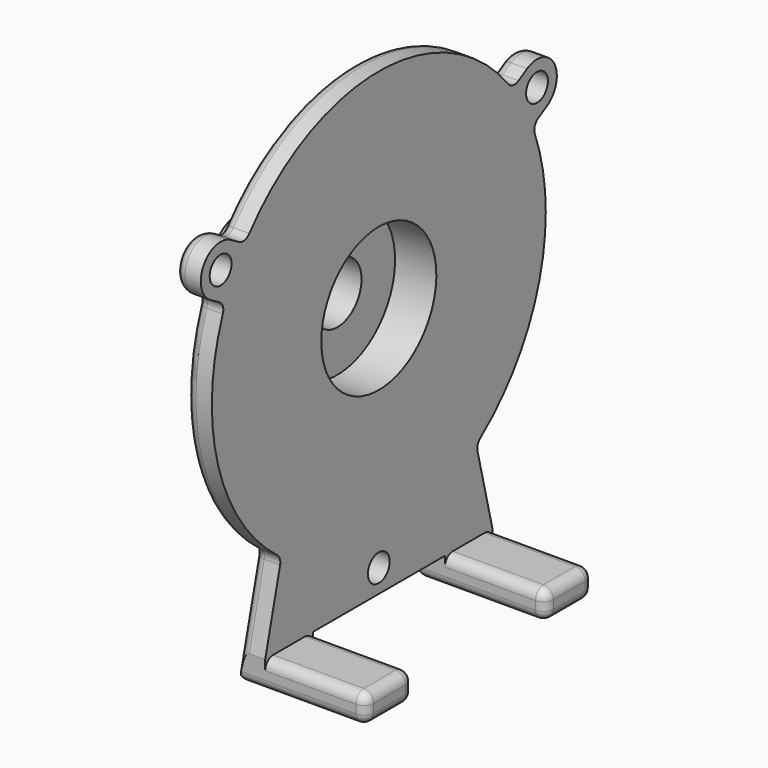
from build123d import *

# Parameters (mm, degrees)
F2_R          = 2.75
F3_DEPTH      = 5.2
F4_DEPTH      = 5.2
F5_DEPTH      = 5.2
F2_W          = 12
F2_H          = 5.7
F6_DEPTH      = 20.28
F6_DEPTH_BACK = 5.2
F7_T1_DEPTH   = 5.2
F7_T3_DEPTH   = 1.7
F7_T5_DEPTH   = 18.28
F7_T7_DEPTH   = 8
F7_T9_DEPTH   = 8
F7_T11_DEPTH  = 28.48
F7_T13_DEPTH  = 22
F7_T15_DEPTH  = 22
F7_S19_W      = 2.04
F7_S19_H      = 2.04
F7_T20_DEPTH  = 2.04
F7_S25_W      = 2.04
F7_S25_H      = 2.04
F7_T26_DEPTH  = 2.04
F7_S31_W      = 2.04
F7_S31_H      = 2.04
F7_T32_DEPTH  = 2.04
F7_S37_W      = 2.04
F7_S37_H      = 2.04
F7_T38_DEPTH  = 2.04
F7_S43_W      = 2.04
F7_S43_H      = 2.04
F7_T44_DEPTH  = 2.04
F7_S49_W      = 2.04
F7_S49_H      = 2.04
F7_T50_DEPTH  = 2.04
F7_S55_W      = 2.04
F7_S55_H      = 2.04
F7_T56_DEPTH  = 2.04
F7_S61_W      = 2.04
F7_S61_H      = 2.04
F7_T62_DEPTH  = 2.04
F7_T69_DEPTH  = 2.5190996878
F7_T71_DEPTH  = 2.5190996878
F7_T73_DEPTH  = 24.1890808372
F7_T75_DEPTH  = 24.1890808372
F7_T77_DEPTH  = 2.5190996878
F7_T79_DEPTH  = 2.5190996878
F7_T82_ANGLE  = 73.3925557793
F7_T84_ANGLE  = 101.7336044326
F7_T86_ANGLE  = 180
F7_T88_ANGLE  = 73.3925557793
F7_T90_ANGLE  = 180
F7_T92_ANGLE  = 80.8668022163
F7_T94_ANGLE  = 80.8668022163
F7_T96_ANGLE  = 66.3959416665
F7_T98_ANGLE  = 66.3959416665
F7_T100_ANGLE = 80.8668022163
F7_T102_ANGLE = 80.8668022163


# Not quite as in the source:
# - a fillet or chamfer that OpenCascade refuses, or shapes differently, is made with other operations: its cross-section is extruded or revolved along the edge and cut away or added


with BuildPart() as f1:
    # F0 (on Front) → F1 (revolve)
    with BuildSketch(Plane.XZ):
        Polygon((0, 14.51), (0, 42.1), (-5.2, 42.1), (-5.2, 20), (-10.9, 20), (-10.9, 8.925), (-28.3, 8.925), (-28.3, 6.05), (-8.33, 6.05), (-8.33, 14.51), align=None)
    revolve(axis=Axis((-6.4437054098, 0, 0), (1, 0, 0)))

    # F2 (on Right) → F3 (join, through all)
    with BuildSketch(Plane.YZ):
        with BuildLine():
            ThreePointArc((-38.7016228918, 16.5708897028), (-36.4596694993, 21.05), (-33.7016228918, 25.2311437406))
            Line((-33.7016228918, 25.2311437406), (-37.3891300983, 27.3601270189))
            ThreePointArc((-37.3891300983, 27.3601270189), (-44.2192571172, 25.53), (-42.3891300983, 18.6998729811))
            Line((-42.3891300983, 18.6998729811), (-38.7016228918, 16.5708897028))
        make_face()
        with Locations((-39.8891300983, 23.03)):
            Circle(F2_R, mode=Mode.SUBTRACT)
    extrude(amount=-F3_DEPTH)

    # F2 (on Right) → F4 (join, through all)
    with BuildSketch(Plane.YZ):
        with BuildLine():
            Line((38.7016228918, 16.5708897028), (42.3891300983, 18.6998729811))
            ThreePointArc((42.3891300983, 18.6998729811), (44.2192571172, 25.53), (37.3891300983, 27.3601270189))
            Line((37.3891300983, 27.3601270189), (33.7016228918, 25.2311437406))
            ThreePointArc((33.7016228918, 25.2311437406), (36.4596694993, 21.05), (38.7016228918, 16.5708897028))
        make_face()
        with Locations((39.8891300983, 23.03)):
            Circle(F2_R, mode=Mode.SUBTRACT)
    extrude(amount=-F4_DEPTH)

    # F2 (on Right) → F5 (join, through all)
    with BuildSketch(Plane.YZ):
        with BuildLine():
            ThreePointArc((24.57, -34.1866216523), (0, -42.1), (-24.57, -34.1866216523))
            Line((-24.57, -34.1866216523), (-28.65, -50.71))
            Line((-28.65, -50.71), (-16.65, -50.71))
            Line((-16.65, -50.71), (16.65, -50.71))
            Line((16.65, -50.71), (28.65, -50.71))
            Line((28.65, -50.71), (24.57, -34.1866216523))
        make_face()
        with Locations((0, -46.06)):
            Circle(F2_R, mode=Mode.SUBTRACT)
    extrude(amount=-F5_DEPTH)

    # F2 (on Right) → F6 (join, two sides)
    with BuildSketch(Plane.YZ) as f6_sk:
        with Locations((-22.65, -53.56)):
            Rectangle(F2_W, F2_H)
        with Locations((22.65, -53.56)):
            Rectangle(F2_W, F2_H)
    extrude(amount=F6_DEPTH)
    extrude(f6_sk.sketch, amount=-F6_DEPTH_BACK)

    # F7: fillet of radius 2 on 39 edges, made by hand

    # F7_s2 → F7_t1 (join)
    with BuildSketch(Plane.YZ.offset(-5.2)):
        with BuildLine():
            ThreePointArc((-32.6561640609, 26.5703772804), (-33.8453407807, 25.8656958459), (-35.207525774, 26.100577175))
            Line((-35.207525774, 26.100577175), (-33.7016228918, 25.2311437406))
            ThreePointArc((-33.7016228918, 25.2311437406), (-33.1856498947, 25.9060348387), (-32.6561640609, 26.5703772804))
        make_face()
        with BuildLine():
            ThreePointArc((-40.207525774, 17.4403231372), (-39.3230200794, 16.3780769929), (-39.3387037435, 14.9958790267))
            ThreePointArc((-39.3387037435, 14.9958790267), (-39.028109229, 15.7865984306), (-38.7016228918, 16.5708897028))
            Line((-38.7016228918, 16.5708897028), (-40.207525774, 17.4403231372))
        make_face()
        with BuildLine():
            ThreePointArc((32.6561640609, 26.5703772804), (33.8453407807, 25.8656958459), (35.207525774, 26.100577175))
            Line((35.207525774, 26.100577175), (33.7016228918, 25.2311437406))
            ThreePointArc((33.7016228918, 25.2311437406), (33.1856498947, 25.9060348387), (32.6561640609, 26.5703772804))
        make_face()
        with BuildLine():
            ThreePointArc((39.3387037435, 14.9958790267), (39.3230200794, 16.3780769929), (40.207525774, 17.4403231372))
            Line((40.207525774, 17.4403231372), (38.7016228918, 16.5708897028))
            ThreePointArc((38.7016228918, 16.5708897028), (39.028109229, 15.7865984306), (39.3387037435, 14.9958790267))
        make_face()
        with BuildLine():
            ThreePointArc((24.8889675585, -35.4783916643), (24.9433690993, -34.3370017965), (25.6138407126, -33.4116920246))
            ThreePointArc((25.6138407126, -33.4116920246), (25.0949117582, -33.8031862973), (24.57, -34.1866216523))
            Line((24.57, -34.1866216523), (24.8889675585, -35.4783916643))
        make_face()
        with BuildLine():
            ThreePointArc((-25.6138407126, -33.4116920246), (-24.9433690993, -34.3370017965), (-24.8889675585, -35.4783916643))
            Line((-24.8889675585, -35.4783916643), (-24.57, -34.1866216523))
            ThreePointArc((-24.57, -34.1866216523), (-25.0949117582, -33.8031862973), (-25.6138407126, -33.4116920246))
        make_face()
    extrude(amount=F7_T1_DEPTH)

    # F7_s4 → F7_t3 (cut)
    with BuildSketch(Plane.XY.offset(-54.41)):
        with BuildLine():
            ThreePointArc((18.28, -28.65), (19.6942135624, -28.0642135624), (20.28, -26.65))
            Line((20.28, -26.65), (20.28, -28.65))
            Line((20.28, -28.65), (18.28, -28.65))
        make_face()
        with BuildLine():
            ThreePointArc((18.28, -16.65), (19.6942135624, -17.2357864376), (20.28, -18.65))
            Line((20.28, -18.65), (20.28, -16.65))
            Line((20.28, -16.65), (18.28, -16.65))
        make_face()
        with BuildLine():
            ThreePointArc((18.28, 16.65), (19.6942135624, 17.2357864376), (20.28, 18.65))
            Line((20.28, 18.65), (20.28, 16.65))
            Line((20.28, 16.65), (18.28, 16.65))
        make_face()
        with BuildLine():
            ThreePointArc((18.28, 28.65), (19.6942135624, 28.0642135624), (20.28, 26.65))
            Line((20.28, 26.65), (20.28, 28.65))
            Line((20.28, 28.65), (18.28, 28.65))
        make_face()
    extrude(amount=F7_T3_DEPTH, mode=Mode.SUBTRACT)

    # F7_s6 → F7_t5 (cut)
    with BuildSketch(Plane.YZ):
        with BuildLine():
            ThreePointArc((-28.65, -52.71), (-28.0642135624, -51.2957864376), (-26.65, -50.71))
            Line((-26.65, -50.71), (-28.65, -50.71))
            Line((-28.65, -50.71), (-28.65, -52.71))
        make_face()
        with BuildLine():
            ThreePointArc((-16.65, -52.71), (-17.2357864376, -51.2957864376), (-18.65, -50.71))
            Line((-18.65, -50.71), (-16.65, -50.71))
            Line((-16.65, -50.71), (-16.65, -52.71))
        make_face()
        with BuildLine():
            ThreePointArc((16.65, -52.71), (17.2357864376, -51.2957864376), (18.65, -50.71))
            Line((18.65, -50.71), (16.65, -50.71))
            Line((16.65, -50.71), (16.65, -52.71))
        make_face()
        with BuildLine():
            ThreePointArc((28.65, -52.71), (28.0642135624, -51.2957864376), (26.65, -50.71))
            Line((26.65, -50.71), (28.65, -50.71))
            Line((28.65, -50.71), (28.65, -52.71))
        make_face()
    extrude(amount=F7_T5_DEPTH, mode=Mode.SUBTRACT)

    # F7_s8 → F7_t7 (cut)
    with BuildSketch(Plane.XZ.offset(18.65)):
        with BuildLine():
            ThreePointArc((18.28, -50.71), (19.6942135624, -51.2957864376), (20.28, -52.71))
            Line((20.28, -52.71), (20.28, -50.71))
            Line((20.28, -50.71), (18.28, -50.71))
        make_face()
        with BuildLine():
            ThreePointArc((18.28, -56.41), (19.6942135624, -55.8242135624), (20.28, -54.41))
            Line((20.28, -54.41), (20.28, -56.41))
            Line((20.28, -56.41), (18.28, -56.41))
        make_face()
    extrude(amount=F7_T7_DEPTH, mode=Mode.SUBTRACT)

    # F7_s10 → F7_t9 (cut)
    with BuildSketch(Plane.XZ.offset(-26.65)):
        with BuildLine():
            ThreePointArc((18.28, -50.71), (19.6942135624, -51.2957864376), (20.28, -52.71))
            Line((20.28, -52.71), (20.28, -50.71))
            Line((20.28, -50.71), (18.28, -50.71))
        make_face()
        with BuildLine():
            ThreePointArc((18.28, -56.41), (19.6942135624, -55.8242135624), (20.28, -54.41))
            Line((20.28, -54.41), (20.28, -56.41))
            Line((20.28, -56.41), (18.28, -56.41))
        make_face()
    extrude(amount=F7_T9_DEPTH, mode=Mode.SUBTRACT)

    # F7_s12 → F7_t11 (cut)
    with BuildSketch(Plane.YZ.offset(-10.2)):
        with BuildLine():
            ThreePointArc((-28.65, -54.41), (-28.0642135624, -55.8242135624), (-26.65, -56.41))
            Line((-26.65, -56.41), (-28.65, -56.41))
            Line((-28.65, -56.41), (-28.65, -54.41))
        make_face()
        with BuildLine():
            ThreePointArc((26.65, -56.41), (28.0642135624, -55.8242135624), (28.65, -54.41))
            Line((28.65, -54.41), (28.65, -56.41))
            Line((28.65, -56.41), (26.65, -56.41))
        make_face()
        with BuildLine():
            ThreePointArc((16.65, -54.41), (17.2357864376, -55.8242135624), (18.65, -56.41))
            Line((18.65, -56.41), (16.65, -56.41))
            Line((16.65, -56.41), (16.65, -54.41))
        make_face()
        with BuildLine():
            ThreePointArc((-18.65, -56.41), (-17.2357864376, -55.8242135624), (-16.65, -54.41))
            Line((-16.65, -54.41), (-16.65, -56.41))
            Line((-16.65, -56.41), (-18.65, -56.41))
        make_face()
    extrude(amount=F7_T11_DEPTH, mode=Mode.SUBTRACT)

    # F7_s14 → F7_t13 (cut)
    with BuildSketch(Plane.XZ.offset(11.65)):
        with BuildLine():
            ThreePointArc((-5.2, -54.41), (-4.6142135624, -55.8242135624), (-3.2, -56.41))
            Line((-3.2, -56.41), (-5.2, -56.41))
            Line((-5.2, -56.41), (-5.2, -54.41))
        make_face()
    extrude(amount=F7_T13_DEPTH, mode=Mode.SUBTRACT)

    # F7_s16 → F7_t15 (cut)
    with BuildSketch(Plane.XZ.offset(-33.65)):
        with BuildLine():
            ThreePointArc((-5.2, -54.41), (-4.6142135624, -55.8242135624), (-3.2, -56.41))
            Line((-3.2, -56.41), (-5.2, -56.41))
            Line((-5.2, -56.41), (-5.2, -54.41))
        make_face()
    extrude(amount=F7_T15_DEPTH, mode=Mode.SUBTRACT)


with BuildPart() as f7_tool18:
    # F7_s19 → F7_t20 (new body)
    with BuildSketch(Plane.YZ.offset(18.28)):
        with Locations((-27.67, -51.69)):
            Rectangle(F7_S19_W, F7_S19_H)
    extrude(amount=F7_T20_DEPTH)

    # F7_s21 → F7_t22 (revolve, cut)
    with BuildSketch(Plane(origin=(18.28, -26.65, -52.71), x_dir=(0, 0.7071067812, -0.7071067812), z_dir=(0, -0.7071067812, -0.7071067812))):
        with BuildLine():
            ThreePointArc((0, -2), (2, 0), (0, 2))
            Line((0, 2), (0, -2))
        make_face()
    revolve(axis=Axis((18.28, -26.65, -52.71), (1, 0, 0)), mode=Mode.SUBTRACT)


with BuildPart() as f1_1:
    add(f1.part)

    # F7_t17: cut F7_tool18
    add(f7_tool18.part, mode=Mode.SUBTRACT)


with BuildPart() as f7_tool24:
    # F7_s25 → F7_t26 (new body)
    with BuildSketch(Plane.XY.offset(-54.41)):
        with Locations((19.3, -27.67)):
            Rectangle(F7_S25_W, F7_S25_H)
    extrude(amount=-F7_T26_DEPTH)

    # F7_s27 → F7_t28 (revolve, cut)
    with BuildSketch(Plane(origin=(18.28, -26.65, -54.41), x_dir=(-0.7071067812, 0.7071067812, 0), z_dir=(-0.7071067812, -0.7071067812, 0))):
        with BuildLine():
            ThreePointArc((0, -2), (2, 0), (0, 2))
            Line((0, 2), (0, -2))
        make_face()
    revolve(axis=Axis((18.28, -26.65, -54.41), (0, 0, -1)), mode=Mode.SUBTRACT)


with BuildPart() as f1_2:
    add(f1_1.part)

    # F7_t23: cut F7_tool24
    add(f7_tool24.part, mode=Mode.SUBTRACT)


with BuildPart() as f7_tool30:
    # F7_s31 → F7_t32 (new body)
    with BuildSketch(Plane.XY.offset(-54.41)):
        with Locations((19.3, -17.63)):
            Rectangle(F7_S31_W, F7_S31_H)
    extrude(amount=-F7_T32_DEPTH)

    # F7_s33 → F7_t34 (revolve, cut)
    with BuildSketch(Plane(origin=(18.28, -18.65, -54.41), x_dir=(-0.7071067812, -0.7071067812, 0), z_dir=(0.7071067812, -0.7071067812, 0))):
        with BuildLine():
            ThreePointArc((0, -2), (2, 0), (0, 2))
            Line((0, 2), (0, -2))
        make_face()
    revolve(axis=Axis((18.28, -18.65, -54.41), (0, 0, -1)), mode=Mode.SUBTRACT)


with BuildPart() as f1_3:
    add(f1_2.part)

    # F7_t29: cut F7_tool30
    add(f7_tool30.part, mode=Mode.SUBTRACT)


with BuildPart() as f7_tool36:
    # F7_s37 → F7_t38 (new body)
    with BuildSketch(Plane.XZ.offset(18.65)):
        with Locations((19.3, -51.69)):
            Rectangle(F7_S37_W, F7_S37_H)
    extrude(amount=-F7_T38_DEPTH)

    # F7_s39 → F7_t40 (revolve, cut)
    with BuildSketch(Plane(origin=(18.28, -18.65, -52.71), x_dir=(-0.7071067812, 0, -0.7071067812), z_dir=(0.7071067812, 0, -0.7071067812))):
        with BuildLine():
            ThreePointArc((0, -2), (2, 0), (0, 2))
            Line((0, 2), (0, -2))
        make_face()
    revolve(axis=Axis((18.28, -18.65, -52.71), (0, 1, 0)), mode=Mode.SUBTRACT)


with BuildPart() as f1_4:
    add(f1_3.part)

    # F7_t35: cut F7_tool36
    add(f7_tool36.part, mode=Mode.SUBTRACT)


with BuildPart() as f7_tool42:
    # F7_s43 → F7_t44 (new body)
    with BuildSketch(Plane.XZ.offset(-18.65)):
        with Locations((19.3, -51.69)):
            Rectangle(F7_S43_W, F7_S43_H)
    extrude(amount=F7_T44_DEPTH)

    # F7_s45 → F7_t46 (revolve, cut)
    with BuildSketch(Plane(origin=(18.28, 18.65, -52.71), x_dir=(-0.7071067812, 0, -0.7071067812), z_dir=(-0.7071067812, 0, 0.7071067812))):
        with BuildLine():
            ThreePointArc((0, -2), (2, 0), (0, 2))
            Line((0, 2), (0, -2))
        make_face()
    revolve(axis=Axis((18.28, 18.65, -52.71), (0, -1, 0)), mode=Mode.SUBTRACT)


with BuildPart() as f1_5:
    add(f1_4.part)

    # F7_t41: cut F7_tool42
    add(f7_tool42.part, mode=Mode.SUBTRACT)


with BuildPart() as f7_tool48:
    # F7_s49 → F7_t50 (new body)
    with BuildSketch(Plane.XZ.offset(-18.65)):
        with Locations((19.3, -55.43)):
            Rectangle(F7_S49_W, F7_S49_H)
    extrude(amount=F7_T50_DEPTH)

    # F7_s51 → F7_t52 (revolve, cut)
    with BuildSketch(Plane(origin=(18.28, 18.65, -54.41), x_dir=(-0.7071067812, 0, 0.7071067812), z_dir=(0.7071067812, 0, 0.7071067812))):
        with BuildLine():
            ThreePointArc((0, -2), (2, 0), (0, 2))
            Line((0, 2), (0, -2))
        make_face()
    revolve(axis=Axis((18.28, 18.65, -54.41), (0, -1, 0)), mode=Mode.SUBTRACT)


with BuildPart() as f1_6:
    add(f1_5.part)

    # F7_t47: cut F7_tool48
    add(f7_tool48.part, mode=Mode.SUBTRACT)


with BuildPart() as f7_tool54:
    # F7_s55 → F7_t56 (new body)
    with BuildSketch(Plane.YZ.offset(18.28)):
        with Locations((27.67, -55.43)):
            Rectangle(F7_S55_W, F7_S55_H)
    extrude(amount=F7_T56_DEPTH)

    # F7_s57 → F7_t58 (revolve, cut)
    with BuildSketch(Plane(origin=(18.28, 26.65, -54.41), x_dir=(0, -0.7071067812, 0.7071067812), z_dir=(0, 0.7071067812, 0.7071067812))):
        with BuildLine():
            ThreePointArc((0, -2), (2, 0), (0, 2))
            Line((0, 2), (0, -2))
        make_face()
    revolve(axis=Axis((18.28, 26.65, -54.41), (1, 0, 0)), mode=Mode.SUBTRACT)


with BuildPart() as f1_7:
    add(f1_6.part)

    # F7_t53: cut F7_tool54
    add(f7_tool54.part, mode=Mode.SUBTRACT)


with BuildPart() as f7_tool60:
    # F7_s61 → F7_t62 (new body)
    with BuildSketch(Plane.YZ.offset(18.28)):
        with Locations((27.67, -51.69)):
            Rectangle(F7_S61_W, F7_S61_H)
    extrude(amount=F7_T62_DEPTH)

    # F7_s63 → F7_t64 (revolve, cut)
    with BuildSketch(Plane(origin=(18.28, 26.65, -52.71), x_dir=(0, -0.7071067812, -0.7071067812), z_dir=(0, -0.7071067812, 0.7071067812))):
        with BuildLine():
            ThreePointArc((0, -2), (2, 0), (0, 2))
            Line((0, 2), (0, -2))
        make_face()
    revolve(axis=Axis((18.28, 26.65, -52.71), (1, 0, 0)), mode=Mode.SUBTRACT)


with BuildPart() as f1_8:
    add(f1_7.part)

    # F7_t59: cut F7_tool60
    add(f7_tool60.part, mode=Mode.SUBTRACT)

    # F7_s65 → F7_t66 (revolve, cut)
    with BuildSketch(Plane.XZ):
        with BuildLine():
            ThreePointArc((-10.9, 18), (-10.3142135624, 19.4142135624), (-8.9, 20))
            Line((-8.9, 20), (-10.9, 20))
            Line((-10.9, 20), (-10.9, 18))
        make_face()
    revolve(axis=Axis((-10.9, 0, 0), (1, 0, 0)), mode=Mode.SUBTRACT)

    # F7_s67 → F7_t68 (revolve, cut)
    with BuildSketch(Plane.XZ):
        with BuildLine():
            ThreePointArc((-28.3, 6.925), (-27.7142135624, 8.3392135624), (-26.3, 8.925))
            Line((-26.3, 8.925), (-28.3, 8.925))
            Line((-28.3, 8.925), (-28.3, 6.925))
        make_face()
    revolve(axis=Axis((-28.3, 0, 0), (1, 0, 0)), mode=Mode.SUBTRACT)

    # F7_s70 → F7_t69 (cut)
    with BuildSketch(Plane(origin=(0, -37.707525774, 21.7704501561), x_dir=(1, 0, 0), z_dir=(0, -0.8660254038, 0.5))):
        with BuildLine():
            ThreePointArc((-3.2, 5), (-4.6142135624, 4.4142135624), (-5.2, 3))
            Line((-5.2, 3), (-5.2, 5))
            Line((-5.2, 5), (-3.2, 5))
        make_face()
    extrude(amount=F7_T69_DEPTH, mode=Mode.SUBTRACT)

    # F7_s72 → F7_t71 (cut)
    with BuildSketch(Plane(origin=(0, -39.8891300983, 23.03), x_dir=(1, 0, 0), z_dir=(0, 0.8660254038, -0.5))):
        with BuildLine():
            ThreePointArc((-3.2, 5), (-4.6142135624, 4.4142135624), (-5.2, 3))
            Line((-5.2, 3), (-5.2, 5))
            Line((-5.2, 5), (-3.2, 5))
        make_face()
    extrude(amount=F7_T71_DEPTH, mode=Mode.SUBTRACT)

    # F7_s74 → F7_t73 (cut)
    with BuildSketch(Plane(origin=(0, -9.6872865146, -39.2320343731), x_dir=(1, 0, 0), z_dir=(0, -0.2397229309, -0.9708413446))):
        with BuildLine():
            ThreePointArc((-3.2, 15.6582546967), (-4.6142135624, 15.072468259), (-5.2, 13.6582546967))
            Line((-5.2, 13.6582546967), (-5.2, 15.6582546967))
            Line((-5.2, 15.6582546967), (-3.2, 15.6582546967))
        make_face()
    extrude(amount=F7_T73_DEPTH, mode=Mode.SUBTRACT)

    # F7_s76 → F7_t75 (cut)
    with BuildSketch(Plane(origin=(0, 15.4859638688, -62.7157941379), x_dir=(1, 0, 0), z_dir=(0, -0.2397229309, 0.9708413446))):
        with BuildLine():
            ThreePointArc((-3.2, 15.6582546967), (-4.6142135624, 15.072468259), (-5.2, 13.6582546967))
            Line((-5.2, 13.6582546967), (-5.2, 15.6582546967))
            Line((-5.2, 15.6582546967), (-3.2, 15.6582546967))
        make_face()
    extrude(amount=F7_T75_DEPTH, mode=Mode.SUBTRACT)

    # F7_s78 → F7_t77 (cut)
    with BuildSketch(Plane(origin=(0, 37.707525774, 21.7704501561), x_dir=(1, 0, 0), z_dir=(0, 0.8660254038, 0.5))):
        with BuildLine():
            ThreePointArc((-3.2, 5), (-4.6142135624, 4.4142135624), (-5.2, 3))
            Line((-5.2, 3), (-5.2, 5))
            Line((-5.2, 5), (-3.2, 5))
        make_face()
    extrude(amount=F7_T77_DEPTH, mode=Mode.SUBTRACT)

    # F7_s80 → F7_t79 (cut)
    with BuildSketch(Plane(origin=(0, 39.8891300983, 23.03), x_dir=(1, 0, 0), z_dir=(0, -0.8660254038, -0.5))):
        with BuildLine():
            ThreePointArc((-3.2, 5), (-4.6142135624, 4.4142135624), (-5.2, 3))
            Line((-5.2, 3), (-5.2, 5))
            Line((-5.2, 5), (-3.2, 5))
        make_face()
    extrude(amount=F7_T79_DEPTH, mode=Mode.SUBTRACT)

    # F7_s81 → F7_t82 (revolve, cut)
    with BuildSketch(Plane(origin=(0, 0, 0), x_dir=(1, 0, 0), z_dir=(0, 0.7936268889, -0.6084047675))):
        with BuildLine():
            ThreePointArc((-3.2, 42.1), (-4.6142135624, 41.5142135624), (-5.2, 40.1))
            Line((-5.2, 40.1), (-5.2, 42.1))
            Line((-5.2, 42.1), (-3.2, 42.1))
        make_face()
    revolve(axis=Axis((-5.2, 0, 0), (-1, 0, 0)), revolution_arc=F7_T82_ANGLE, mode=Mode.SUBTRACT)

    # F7_s83 → F7_t84 (revolve, cut)
    with BuildSketch(Plane(origin=(0, 0, 0), x_dir=(1, 0, 0), z_dir=(0, -0.6311253511, -0.7756808566))):
        with BuildLine():
            ThreePointArc((-3.2, 42.1), (-4.6142135624, 41.5142135624), (-5.2, 40.1))
            Line((-5.2, 40.1), (-5.2, 42.1))
            Line((-5.2, 42.1), (-3.2, 42.1))
        make_face()
    revolve(axis=Axis((-5.2, 0, 0), (-1, 0, 0)), revolution_arc=F7_T84_ANGLE, mode=Mode.SUBTRACT)

    # F7_s85 → F7_t86 (revolve, cut)
    with BuildSketch(Plane(origin=(0, -39.8891300983, 23.03), x_dir=(1, 0, 0), z_dir=(0, 0.8660254038, -0.5))):
        with BuildLine():
            ThreePointArc((-3.2, -5), (-4.6142135624, -4.4142135624), (-5.2, -3))
            Line((-5.2, -3), (-5.2, -5))
            Line((-5.2, -5), (-3.2, -5))
        make_face()
    revolve(axis=Axis((-5.2, -39.8891300983, 23.03), (1, 0, 0)), revolution_arc=F7_T86_ANGLE, mode=Mode.SUBTRACT)

    # F7_s87 → F7_t88 (revolve, cut)
    with BuildSketch(Plane(origin=(0, 0, 0), x_dir=(1, 0, 0), z_dir=(0, -0.3561966515, 0.9344110153))):
        with BuildLine():
            ThreePointArc((-3.2, 42.1), (-4.6142135624, 41.5142135624), (-5.2, 40.1))
            Line((-5.2, 40.1), (-5.2, 42.1))
            Line((-5.2, 42.1), (-3.2, 42.1))
        make_face()
    revolve(axis=Axis((-5.2, 0, 0), (-1, 0, 0)), revolution_arc=F7_T88_ANGLE, mode=Mode.SUBTRACT)

    # F7_s89 → F7_t90 (revolve, cut)
    with BuildSketch(Plane(origin=(0, 39.8891300983, 23.03), x_dir=(1, 0, 0), z_dir=(0, -0.8660254038, -0.5))):
        with BuildLine():
            ThreePointArc((-3.2, -5), (-4.6142135624, -4.4142135624), (-5.2, -3))
            Line((-5.2, -3), (-5.2, -5))
            Line((-5.2, -5), (-3.2, -5))
        make_face()
    revolve(axis=Axis((-5.2, 39.8891300983, 23.03), (1, 0, 0)), revolution_arc=F7_T90_ANGLE, mode=Mode.SUBTRACT)

    # F7_s91 → F7_t92 (revolve, cut)
    with BuildSketch(Plane(origin=(0, 0, 0), x_dir=(1, 0, 0), z_dir=(0, -0.6311253511, 0.7756808566))):
        with BuildLine():
            ThreePointArc((-3.2, 42.1), (-4.6142135624, 41.5142135624), (-5.2, 40.1))
            Line((-5.2, 40.1), (-5.2, 42.1))
            Line((-5.2, 42.1), (-3.2, 42.1))
        make_face()
    revolve(axis=Axis((-5.2, 34.207525774, 27.8326279826), (1, 0, 0)), revolution_arc=F7_T92_ANGLE, mode=Mode.SUBTRACT)

    # F7_s93 → F7_t94 (revolve, cut)
    with BuildSketch(Plane(origin=(0, 0, 0), x_dir=(1, 0, 0), z_dir=(0, 0.3561966515, -0.9344110153))):
        with BuildLine():
            ThreePointArc((-3.2, -42.1), (-4.6142135624, -41.5142135624), (-5.2, -40.1))
            Line((-5.2, -40.1), (-5.2, -42.1))
            Line((-5.2, -42.1), (-3.2, -42.1))
        make_face()
    revolve(axis=Axis((-5.2, 41.207525774, 15.7082723296), (-1, 0, 0)), revolution_arc=F7_T94_ANGLE, mode=Mode.SUBTRACT)

    # F7_s95 → F7_t96 (revolve, cut)
    with BuildSketch(Plane(origin=(0, 9.6872865146, -39.2320343731), x_dir=(1, 0, 0), z_dir=(0, 0.2397229309, -0.9708413446))):
        with BuildLine():
            ThreePointArc((-3.2, -15.6582546967), (-4.6142135624, -15.072468259), (-5.2, -13.6582546967))
            Line((-5.2, -13.6582546967), (-5.2, -15.6582546967))
            Line((-5.2, -15.6582546967), (-3.2, -15.6582546967))
        make_face()
    revolve(axis=Axis((-5.2, 26.8306502477, -34.9989458025), (-1, 0, 0)), revolution_arc=F7_T96_ANGLE, mode=Mode.SUBTRACT)

    # F7_s97 → F7_t98 (revolve, cut)
    with BuildSketch(Plane(origin=(0, 0, 0), x_dir=(1, 0, 0), z_dir=(0, -0.7936268889, 0.6084047675))):
        with BuildLine():
            ThreePointArc((-3.2, -42.1), (-4.6142135624, -41.5142135624), (-5.2, -40.1))
            Line((-5.2, -40.1), (-5.2, -42.1))
            Line((-5.2, -42.1), (-3.2, -42.1))
        make_face()
    revolve(axis=Axis((-5.2, -26.8306502477, -34.9989458025), (-1, 0, 0)), revolution_arc=F7_T98_ANGLE, mode=Mode.SUBTRACT)

    # F7_s99 → F7_t100 (revolve, cut)
    with BuildSketch(Plane(origin=(0, -37.707525774, 21.7704501561), x_dir=(1, 0, 0), z_dir=(0, -0.8660254038, 0.5))):
        with BuildLine():
            ThreePointArc((-3.2, -5), (-4.6142135624, -4.4142135624), (-5.2, -3))
            Line((-5.2, -3), (-5.2, -5))
            Line((-5.2, -5), (-3.2, -5))
        make_face()
    revolve(axis=Axis((-5.2, -41.207525774, 15.7082723296), (-1, 0, 0)), revolution_arc=F7_T100_ANGLE, mode=Mode.SUBTRACT)

    # F7_s101 → F7_t102 (revolve, cut)
    with BuildSketch(Plane(origin=(0, 0, 0), x_dir=(1, 0, 0), z_dir=(0, 0.6311253511, 0.7756808566))):
        with BuildLine():
            ThreePointArc((-3.2, -42.1), (-4.6142135624, -41.5142135624), (-5.2, -40.1))
            Line((-5.2, -40.1), (-5.2, -42.1))
            Line((-5.2, -42.1), (-3.2, -42.1))
        make_face()
    revolve(axis=Axis((-5.2, -34.207525774, 27.8326279826), (-1, 0, 0)), revolution_arc=F7_T102_ANGLE, mode=Mode.SUBTRACT)


solid = f1_8.part
